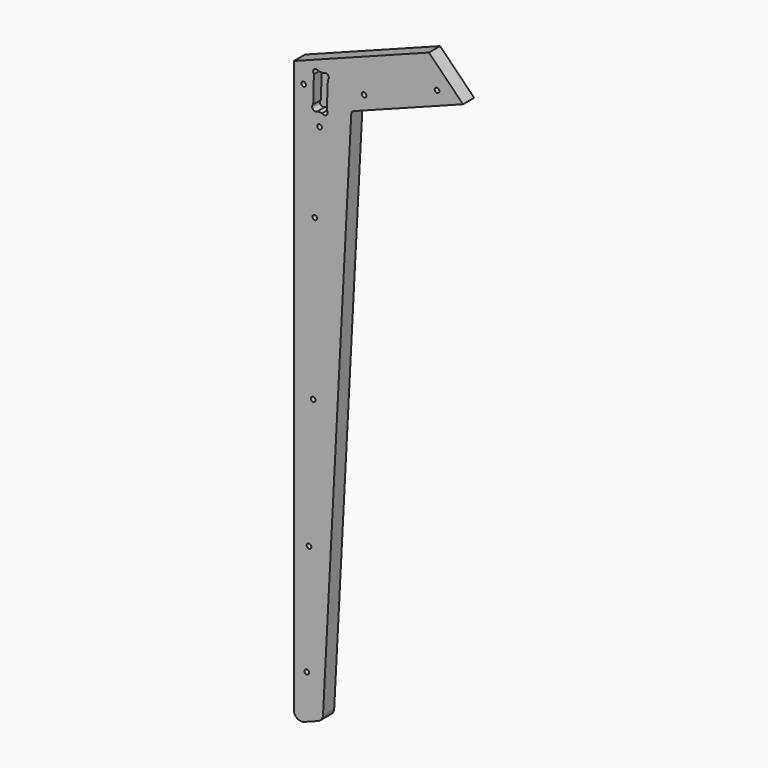
from build123d import *

# Parameters (mm, degrees)
F0_R     = 3
F1_DEPTH = 18
F2_DEPTH = 14
F3_DEPTH = 12.5


# Not quite as in the source:
# - ends of sketch curves that miss each other by under 0.0002 mm in the source are joined


with BuildPart() as f1:
    # F0 (on Front) → F1 (new body)
    with BuildSketch(Plane.XZ):
        with BuildLine():
            Line((-119.3285324557, -448.2617723394), (-101.6685144557, -441.5452453394))
            ThreePointArc((-101.6685144557, -441.5452453394), (-97.1422559669, -438.0887567531), (-95.2370421293, -432.7217753041))
            Line((-95.2370421293, -432.7217753041), (-58.8235234557, 262.0895416606))
            ThreePointArc((-58.8235234557, 262.0895416606), (-58.06143799, 264.2363343101), (-56.250934498, 265.6189297718))
            Line((-56.250934498, 265.6189297718), (85.2578445443, 319.4380986606))
            Line((85.2578445443, 319.4380986606), (41.3370915443, 363.9049416606))
            Line((41.3370915443, 363.9049416606), (-132.8833544557, 297.6447436606))
            Line((-132.8833544557, 297.6447436606), (-132.8833544557, -438.9149423394))
            ThreePointArc((-132.8833544557, -438.9149423394), (-128.5601395631, -447.1474456551), (-119.3285324557, -448.2617723394))
        make_face()
        with Locations((-116.1363294557, -390.4994083394)):
            Circle(F0_R, mode=Mode.SUBTRACT)
        with Locations((-113.3511164557, -246.7075803394)):
            Circle(F0_R, mode=Mode.SUBTRACT)
        with Locations((-107.9187374557, -78.3756793394)):
            Circle(F0_R, mode=Mode.SUBTRACT)
        with Locations((-105.9467734557, 128.6347116606)):
            Circle(F0_R, mode=Mode.SUBTRACT)
        with Locations((-99.7011464557, 233.7480486606)):
            Circle(F0_R, mode=Mode.SUBTRACT)
        with Locations((-120.2235504557, 275.4892296606)):
            Circle(F0_R, mode=Mode.SUBTRACT)
        with BuildLine():
            ThreePointArc((-90.3754553764, 255.7239337355), (-90.5472879726, 250.0640248228), (-96.2068413545, 250.2471937553))
            Line((-96.2068413545, 250.2471937553), (-102.4861304557, 250.4567146606))
            ThreePointArc((-102.4861304557, 250.4567146606), (-108.1617141765, 250.6689360163), (-107.9038666822, 256.3426299107))
            Line((-107.9038666822, 256.3426299107), (-107.0299454557, 291.0352376606))
            ThreePointArc((-107.0299454557, 291.0352376606), (-106.7545815371, 296.6558621202), (-101.1313975225, 296.4389595982))
            Line((-101.1313975225, 296.4389595982), (-94.4508164557, 296.2088706606))
            ThreePointArc((-94.4508164557, 296.2088706606), (-88.7851572097, 296.0073908544), (-89.0114747479, 290.3426689785))
            Line((-89.0114747479, 290.3426689785), (-90.3754553764, 255.7239337355))
        make_face(mode=Mode.SUBTRACT)
        with Locations((-42.3545774557, 288.6199666606)):
            Circle(F0_R, mode=Mode.SUBTRACT)
        with Locations((51.7271015443, 324.4037386606)):
            Circle(F0_R, mode=Mode.SUBTRACT)
        with Locations((-116.1363294557, -390.4994083394)):
            Circle(F0_R)
        with Locations((-113.3511164557, -246.7075803394)):
            Circle(F0_R)
        with Locations((-107.9187374557, -78.3756793394)):
            Circle(F0_R)
        with Locations((-105.9467734557, 128.6347116606)):
            Circle(F0_R)
        with Locations((-120.2235504557, 275.4892296606)):
            Circle(F0_R)
        with Locations((-99.7011464557, 233.7480486606)):
            Circle(F0_R)
        with Locations((-42.3545774557, 288.6199666606)):
            Circle(F0_R)
        with Locations((51.7271015443, 324.4037386606)):
            Circle(F0_R)
        with BuildLine():
            Line((-102.4861304557, 250.4567146606), (-96.2068414557, 250.2471936606))
            ThreePointArc((-96.2068414557, 250.2471936606), (-90.5472879726, 250.0640248228), (-90.3754553764, 255.7239337355))
            Line((-90.3754553764, 255.7239337355), (-89.0114744557, 290.3426686606))
            ThreePointArc((-89.0114744557, 290.3426686606), (-88.7851572097, 296.0073908544), (-94.4508168599, 296.2088710928))
            Line((-94.4508168599, 296.2088710928), (-101.1313974557, 296.4389596606))
            ThreePointArc((-101.1313974557, 296.4389596606), (-106.7545815371, 296.6558621202), (-107.0299455087, 291.0352376131))
            Line((-107.0299455087, 291.0352376131), (-107.9038664557, 256.3426296606))
            ThreePointArc((-107.9038664557, 256.3426296606), (-108.1617141765, 250.6689360163), (-102.4861304557, 250.4567146606))
        make_face()
    extrude(amount=-F1_DEPTH)

    # F0 (on Front) → F2 (cut)
    with BuildSketch(Plane.XZ):
        with Locations((-116.1363294557, -390.4994083394)):
            Circle(F0_R)
        with Locations((-113.3511164557, -246.7075803394)):
            Circle(F0_R)
        with Locations((-107.9187374557, -78.3756793394)):
            Circle(F0_R)
        with Locations((-105.9467734557, 128.6347116606)):
            Circle(F0_R)
        with Locations((-120.2235504557, 275.4892296606)):
            Circle(F0_R)
        with Locations((-99.7011464557, 233.7480486606)):
            Circle(F0_R)
        with Locations((-42.3545774557, 288.6199666606)):
            Circle(F0_R)
        with Locations((51.7271015443, 324.4037386606)):
            Circle(F0_R)
    extrude(amount=-F2_DEPTH, mode=Mode.SUBTRACT)

    # F0 (on Front) → F3 (cut)
    with BuildSketch(Plane.XZ):
        with BuildLine():
            Line((-102.4861304557, 250.4567146606), (-96.2068414557, 250.2471936606))
            ThreePointArc((-96.2068414557, 250.2471936606), (-90.5472879726, 250.0640248228), (-90.3754553764, 255.7239337355))
            Line((-90.3754553764, 255.7239337355), (-89.0114744557, 290.3426686606))
            ThreePointArc((-89.0114744557, 290.3426686606), (-88.7851572097, 296.0073908544), (-94.4508168599, 296.2088710928))
            Line((-94.4508168599, 296.2088710928), (-101.1313974557, 296.4389596606))
            ThreePointArc((-101.1313974557, 296.4389596606), (-106.7545815371, 296.6558621202), (-107.0299455087, 291.0352376131))
            Line((-107.0299455087, 291.0352376131), (-107.9038664557, 256.3426296606))
            ThreePointArc((-107.9038664557, 256.3426296606), (-108.1617141765, 250.6689360163), (-102.4861304557, 250.4567146606))
        make_face()
    extrude(amount=-F3_DEPTH, mode=Mode.SUBTRACT)


solid = f1.part
